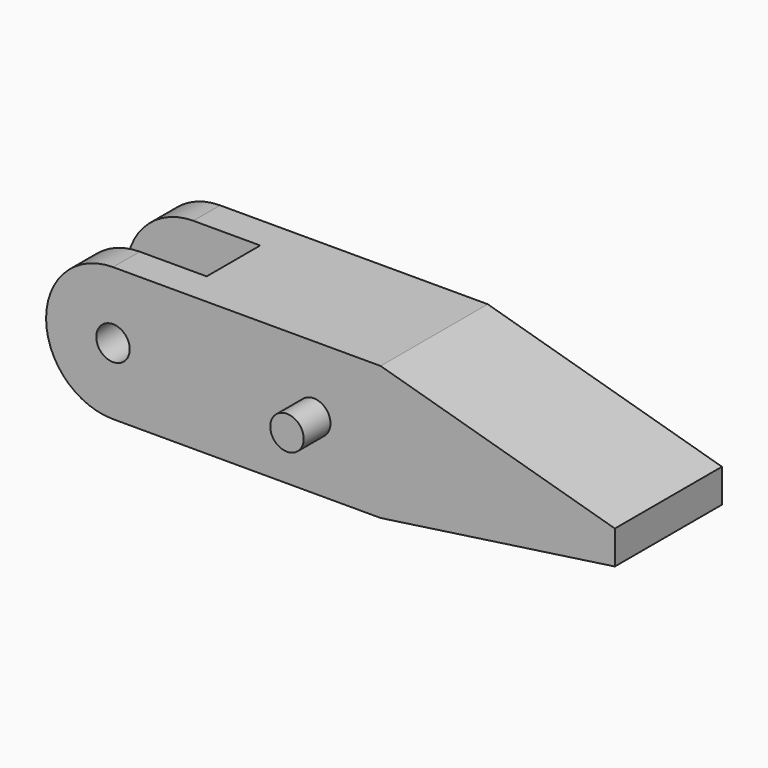
from build123d import *

# Parameters (mm, degrees)
F0_W      = 40
F0_H      = 40
F1_DEPTH  = 80
F2_W      = 10
F2_H      = 40
F3_DEPTH  = 40
F4_R      = 19.99999
F5_R      = 5
F6_DEPTH  = 40.001
F7_R      = 5
F8_DEPTH  = 30
F9_W      = 40
F9_H      = 40
F10_DEPTH = 50
F12_DEPTH = 50.001


# Not quite as in the source:
# - a fillet or chamfer is up to 0.001 mm smaller than in the source, because OpenCascade refuses the exact size


with BuildPart() as f1:
    # F0 (on Right) → F1 (new body)
    with BuildSketch(Plane.YZ):
        Rectangle(F0_W, F0_H)
    extrude(amount=F1_DEPTH)

    # F2 (on face) → F3 (join)
    with BuildSketch(Plane(origin=(0, 0, 0), x_dir=(0, -1, 0), z_dir=(-1, 0, 0))):
        with Locations((15, 0)):
            Rectangle(F2_W, F2_H)
        with Locations((-15, 0)):
            Rectangle(F2_W, F2_H)
    extrude(amount=F3_DEPTH)

    # F4 (radius 20 in the source; OpenCascade refuses exactly that, so slightly less here)
    f4_edges = [f1.edges().sort_by_distance(p)[0] for p in [
        (-40, 15, 20),
        (-40, 15, -20),
        (-40, -15, 20),
        (-40, -15, -20),
    ]]
    fillet(f4_edges, radius=F4_R)

    # F5 (on face) → F6 (cut, through all)
    with BuildSketch(Plane.XZ.offset(20)):
        with Locations((-20, 0)):
            Circle(F5_R)
    extrude(amount=-F6_DEPTH, mode=Mode.SUBTRACT)

    # F7 (on Front) → F8 (join, symmetric)
    with BuildSketch(Plane.XZ):
        with Locations((40, 0)):
            Circle(F7_R)
    extrude(amount=F8_DEPTH, both=True)

    # F9 (on face) → F10 (join)
    with BuildSketch(Plane.YZ.offset(80)):
        Rectangle(F9_W, F9_H)
    extrude(amount=F10_DEPTH)

    # F11 (on face) → F12 (cut, through all)
    with BuildSketch(Plane.XZ.offset(20)):
        Polygon((60, 20), (130, 0), (130, 20), align=None)
        Polygon((130, -20), (130, -10), (60, -20), align=None)
    extrude(amount=-F12_DEPTH, mode=Mode.SUBTRACT)


solid = f1.part
